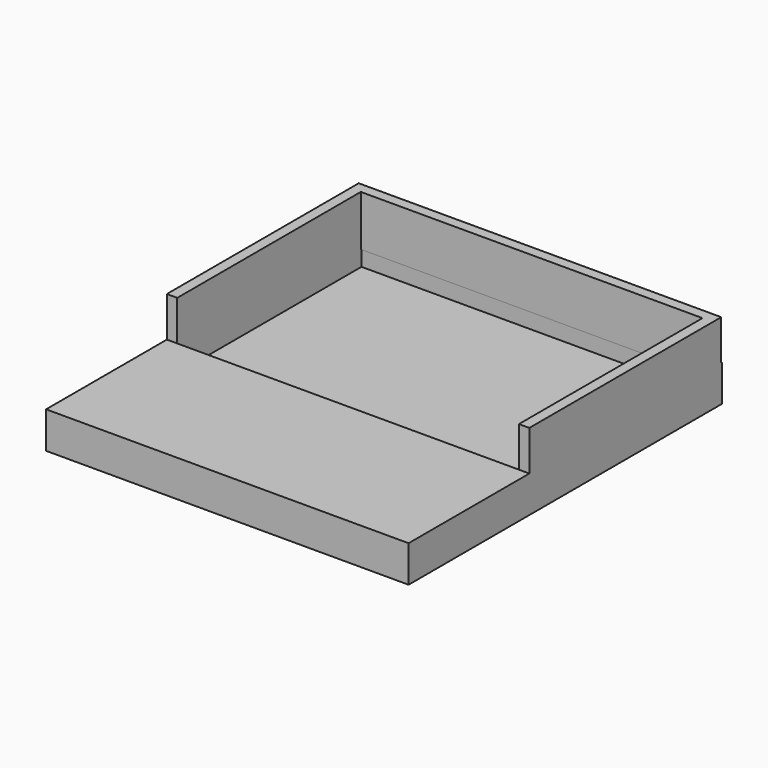
from build123d import *

# Parameters (mm, degrees)
F0_W          = 87
F0_H          = 8.7780428881
F1_DEPTH      = 47
F1_DEPTH_BACK = 47
F2_W          = 57.5710088015
F2_H          = 14.0236988664
F3_DEPTH      = 43.5
F3_DEPTH_BACK = 43.5
F4_T          = 2.5
F4_T3_DEPTH   = 92


# Not quite as in the source:
# - a shell that OpenCascade refuses in one call is made with other operations: the cavity is built on its own and cut out
# - the program builds the solid bodies; features that only make, move or delete a surface that nothing else refers to are left out


with BuildPart() as f1:
    # F0 (on Front) → F1 (new body, two sides)
    with BuildSketch(Plane.XZ) as f1_sk:
        Rectangle(F0_W, F0_H)
    extrude(amount=F1_DEPTH)
    extrude(f1_sk.sketch, amount=-F1_DEPTH_BACK)

    # F2 (on Right) → F3 (join, two sides)
    with BuildSketch(Plane.YZ) as f3_sk:
        with Locations((18.0093571544, 7.0118494332)):
            Rectangle(F2_W, F2_H)
    extrude(amount=F3_DEPTH)
    extrude(f3_sk.sketch, amount=-F3_DEPTH_BACK)

    # F4: shell of thickness 2.5, made by hand


with BuildPart() as f4_core1:
    # F4_t2: copy of F1
    add(f1.part)

    # the walls: a layer under each face that stays
    f4_faces = [f4_core1.faces().sort_by_distance(p)[0] for p in [
        (-43.5, 0, 4.8173387112),
        (0, -28.8880736232, 4.3890214441),
        (0, 46.8974307775, 4.3890214441),
        (0, 47, 0),
        (0, 0, -4.3890214441),
        (0, -47, 0),
        (43.5, 0, 4.8173387112),
        (0, 46.7948615551, 9.2063601552),
    ]]
    thicken(f4_faces, amount=-F4_T, mode=Mode.SUBTRACT)

    # F4_s4 → F4_t3 (cut)
    with BuildSketch(Plane.YZ.offset(-46)):
        Polygon((46.8198615551, 4.4140214441), (46.7948615551, 1.8890214441), (44.2948615551, 1.8890214441), (44.2948615551, 4.3890214441), align=None)
    extrude(amount=F4_T3_DEPTH, mode=Mode.SUBTRACT)


with BuildPart() as f1_1:
    add(f1.part)

    # what is left inside the walls is the cavity
    f4_cavity = [f4_core1.part.solids().sort_by_distance(p)[0] for p in [
        (0, -14.833333, -1.864021),
    ]]
    add(f4_cavity, mode=Mode.SUBTRACT)


solid = f1_1.part
